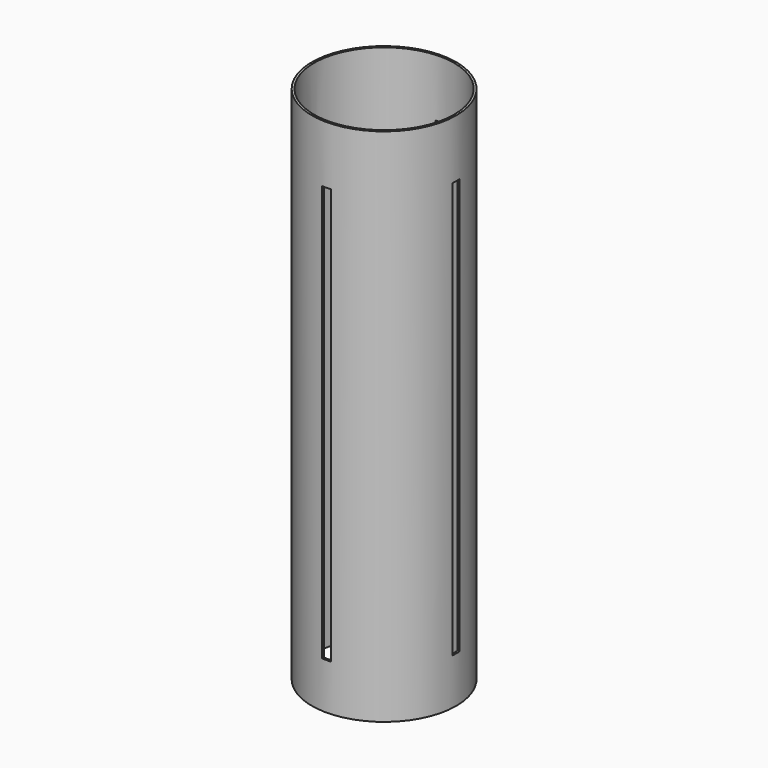
from build123d import *

# Parameters (mm, degrees)
F0_R      = 25
F0_R_2    = 24.25
F1_DEPTH  = 180
F2_W      = 6.5743785797
F2_H      = 144
F2_W_2    = 7.4769609538
F3_DEPTH  = 1.5
F4_DEPTH  = 4
F5_DEPTH  = 4
F6_W      = 7.290615557
F6_H      = 144
F6_W_2    = 7.1577106116
F7_DEPTH  = 1.5
F8_DEPTH  = 4
F9_DEPTH  = 25
F10_DEPTH = 10


# Not quite as in the source:
# - a feature names something its author has since deleted; it is built from what else it names


with BuildPart() as f1:
    # F0 (on Top) → F1 (new body)
    with BuildSketch(Plane.XY):
        Circle(F0_R)
        Circle(F0_R_2, mode=Mode.SUBTRACT)
    extrude(amount=F1_DEPTH)

    # F2 (on Right) → F3 (cut, symmetric)
    with BuildSketch(Plane.YZ):
        with Locations((-28.224690467, 88)):
            Rectangle(F2_W, F2_H)
        with Locations((28.6692082882, 88)):
            Rectangle(F2_W_2, F2_H)
    extrude(amount=F3_DEPTH, both=True, mode=Mode.SUBTRACT)

    # F4 (cut): faces of the model
    f4_faces = [f1.faces().sort_by_distance(p)[0] for p in [
        (0, -24.9375011772, 88),
        (0, 24.9307278113, 88),
    ]]
    extrude(f4_faces, amount=-F4_DEPTH, dir=(0, -1, 0), mode=Mode.SUBTRACT)

    # F5 (cut): a face of the model
    f5_faces = [f1.faces().sort_by_distance(p)[0] for p in [
        (0, 24.9307278113, 88),
    ]]
    extrude(f5_faces, amount=-F5_DEPTH, mode=Mode.SUBTRACT)

    # F6 (on Front) → F7 (join, symmetric)
    with BuildSketch(Plane.XZ):
        with Locations((28.4072192601, 88)):
            Rectangle(F6_W, F6_H)
        with Locations((-28.2881861775, 88)):
            Rectangle(F6_W_2, F6_H)
    extrude(amount=F7_DEPTH, both=True)

    # F8 (cut): faces of the model
    f8_faces = [f1.faces().sort_by_distance(p)[0] for p in [
        (32.0525270386, 0, 88),
        (-31.8670414833, 0, 88),
    ]]
    extrude(f8_faces, amount=-F8_DEPTH, dir=(1, 0, 0), mode=Mode.SUBTRACT)

    # F9 (cut): a face of the model
    f9_faces = [f1.faces().sort_by_distance(p)[0] for p in [
        (28.0525270386, 0, 88),
    ]]
    extrude(f9_faces, amount=-F9_DEPTH, mode=Mode.SUBTRACT)

    # F10 (cut): a face of the model
    f10_faces = [f1.faces().sort_by_distance(p)[0] for p in [
        (-31.8670414833, 0, 88),
    ]]
    extrude(f10_faces, amount=-F10_DEPTH, mode=Mode.SUBTRACT)


solid = f1.part
